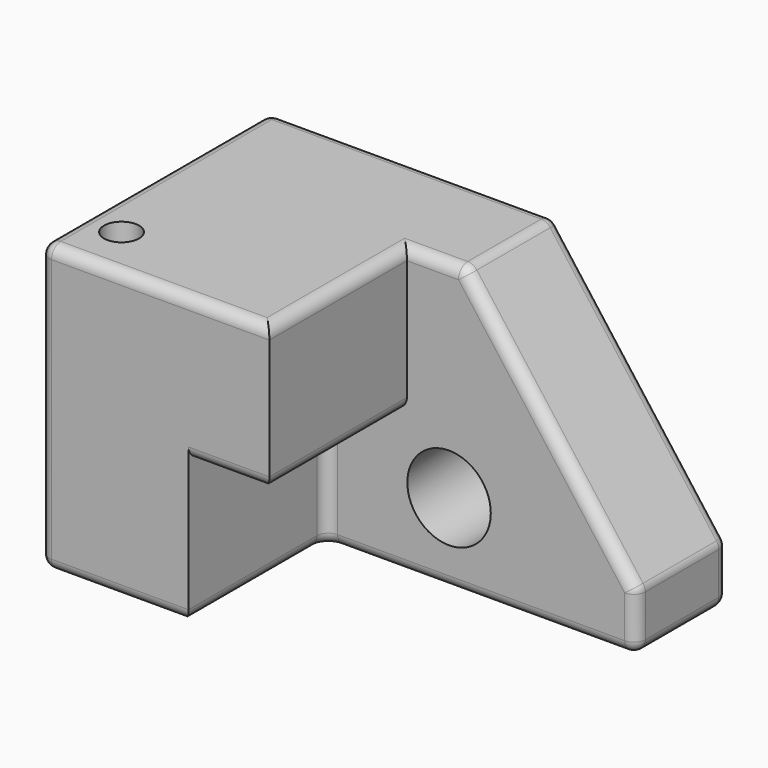
from build123d import *

# Parameters (mm, degrees)
F0_W         = 203.2
F0_H         = 127
F1_DEPTH     = 127
F3_DEPTH     = 76.2
F4_SIZE2     = 101.6
F4_SIZE      = 76.2
F5_R         = 5.08
F6_T1_DEPTH  = 116.84
F6_T3_DEPTH  = 116.84
F6_T5_DEPTH  = 193.04
F6_S9_W      = 5.08
F6_S9_H      = 5.08
F6_T10_DEPTH = 5.08
F6_S15_W     = 5.08
F6_S15_H     = 5.08
F6_T16_DEPTH = 5.08
F6_S21_W     = 5.08
F6_S21_H     = 5.08
F6_T22_DEPTH = 5.08
F6_S27_W     = 5.08
F6_S27_H     = 5.08
F6_T28_DEPTH = 5.08
F7_R         = 18.4939106261
F8_DEPTH     = 50.8
F9_R         = 7.7650869993
F10_DEPTH    = 127


# Not quite as in the source:
# - a fillet or chamfer that OpenCascade refuses, or shapes differently, is made with other operations: its cross-section is extruded or revolved along the edge and cut away or added


with BuildPart() as f1:
    # F0 (on Front) → F1 (new body)
    with BuildSketch(Plane.XZ):
        Rectangle(F0_W, F0_H)
    extrude(amount=F1_DEPTH)

    # F2 (on face) → F3 (cut)
    with BuildSketch(Plane.XZ.offset(127)):
        Polygon((101.6, 63.5), (0, 63.5), (0, 0), (-35.8415916562, 0), (-35.8415916562, -63.5), (101.6, -63.5), align=None)
    extrude(amount=-F3_DEPTH, mode=Mode.SUBTRACT)

    # F4
    f4_edges = [f1.edges().sort_by_distance(p)[0] for p in [
        (101.6, -25.4, 63.5),
    ]]
    f4_side = f1.faces().sort_by_distance((-21.771429, -52.614286, 63.5))[0]
    chamfer(f4_edges, length=F4_SIZE, length2=F4_SIZE2, reference=f4_side)

    # F5
    f5_edges = [f1.edges().sort_by_distance(p)[0] for p in [
        (-101.6, -63.5, 63.5),
        (-50.8, -127, 63.5),
        (0, -88.9, 63.5),
        (12.7, -50.8, 63.5),
        (25.4, -25.4, 63.5),
        (-38.1, 0, 63.5),
        (-17.920796, -127, 0),
        (0, -88.9, 0),
        (-101.6, -127, 0),
        (-68.720796, -127, -63.5),
        (-35.841592, -88.9, -63.5),
        (-35.841592, -50.8, -31.75),
        (32.879204, -50.8, -63.5),
        (101.6, -50.8, -50.8),
        (101.6, -25.4, -63.5),
        (101.6, 0, -50.8),
        (101.6, -25.4, -38.1),
        (63.5, -50.8, 12.7),
        (63.5, 0, 12.7),
    ]]
    fillet(f5_edges, radius=F5_R)

    # F6: fillet of radius 5.08 on 3 edges, made by hand

    # F6_s2 → F6_t1 (cut)
    with BuildSketch(Plane.XZ.offset(5.08)):
        with BuildLine():
            ThreePointArc((-96.52, -63.5), (-100.1121024484, -62.0121024484), (-101.6, -58.42))
            Line((-101.6, -58.42), (-101.6, -63.5))
            Line((-101.6, -63.5), (-96.52, -63.5))
        make_face()
    extrude(amount=F6_T1_DEPTH, mode=Mode.SUBTRACT)

    # F6_s4 → F6_t3 (cut)
    with BuildSketch(Plane.XY.offset(-58.42)):
        with BuildLine():
            ThreePointArc((-96.52, 0), (-100.1121024484, -1.4878975516), (-101.6, -5.08))
            Line((-101.6, -5.08), (-101.6, 0))
            Line((-101.6, 0), (-96.52, 0))
        make_face()
    extrude(amount=F6_T3_DEPTH, mode=Mode.SUBTRACT)

    # F6_s6 → F6_t5 (cut)
    with BuildSketch(Plane.YZ.offset(-96.52)):
        with BuildLine():
            ThreePointArc((0, -58.42), (-1.4878975516, -62.0121024484), (-5.08, -63.5))
            Line((-5.08, -63.5), (0, -63.5))
            Line((0, -63.5), (0, -58.42))
        make_face()
    extrude(amount=F6_T5_DEPTH, mode=Mode.SUBTRACT)


with BuildPart() as f6_tool8:
    # F6_s9 → F6_t10 (new body)
    with BuildSketch(Plane.XZ.offset(5.08)):
        with Locations((99.06, -60.96)):
            Rectangle(F6_S9_W, F6_S9_H)
    extrude(amount=-F6_T10_DEPTH)

    # F6_s11 → F6_t12 (revolve, cut)
    with BuildSketch(Plane(origin=(96.52, -5.08, -58.42), x_dir=(-0.7071067812, 0, 0.7071067812), z_dir=(-0.7071067812, 0, -0.7071067812))):
        with BuildLine():
            ThreePointArc((0, -5.08), (5.08, 0), (0, 5.08))
            Line((0, 5.08), (0, -5.08))
        make_face()
    revolve(axis=Axis((96.52, -5.08, -58.42), (0, 1, 0)), mode=Mode.SUBTRACT)


with BuildPart() as f1_1:
    add(f1.part)

    # F6_t7: cut F6_tool8
    add(f6_tool8.part, mode=Mode.SUBTRACT)


with BuildPart() as f6_tool14:
    # F6_s15 → F6_t16 (new body)
    with BuildSketch(Plane.XZ.offset(5.08)):
        with Locations((-99.06, 60.96)):
            Rectangle(F6_S15_W, F6_S15_H)
    extrude(amount=-F6_T16_DEPTH)

    # F6_s17 → F6_t18 (revolve, cut)
    with BuildSketch(Plane(origin=(-96.52, -5.08, 58.42), x_dir=(0.7071067812, 0, -0.7071067812), z_dir=(0.7071067812, 0, 0.7071067812))):
        with BuildLine():
            ThreePointArc((0, -5.08), (5.08, 0), (0, 5.08))
            Line((0, 5.08), (0, -5.08))
        make_face()
    revolve(axis=Axis((-96.52, -5.08, 58.42), (0, 1, 0)), mode=Mode.SUBTRACT)


with BuildPart() as f1_2:
    add(f1_1.part)

    # F6_t13: cut F6_tool14
    add(f6_tool14.part, mode=Mode.SUBTRACT)


with BuildPart() as f6_tool20:
    # F6_s21 → F6_t22 (new body)
    with BuildSketch(Plane.XY.offset(-58.42)):
        with Locations((-99.06, -124.46)):
            Rectangle(F6_S21_W, F6_S21_H)
    extrude(amount=-F6_T22_DEPTH)

    # F6_s23 → F6_t24 (revolve, cut)
    with BuildSketch(Plane(origin=(-96.52, -121.92, -58.42), x_dir=(0.7071067812, 0.7071067812, 0), z_dir=(-0.7071067812, 0.7071067812, 0))):
        with BuildLine():
            ThreePointArc((0, -5.08), (5.08, 0), (0, 5.08))
            Line((0, 5.08), (0, -5.08))
        make_face()
    revolve(axis=Axis((-96.52, -121.92, -58.42), (0, 0, -1)), mode=Mode.SUBTRACT)


with BuildPart() as f1_3:
    add(f1_2.part)

    # F6_t19: cut F6_tool20
    add(f6_tool20.part, mode=Mode.SUBTRACT)


with BuildPart() as f6_tool26:
    # F6_s27 → F6_t28 (new body)
    with BuildSketch(Plane.XZ.offset(5.08)):
        with Locations((-99.06, -60.96)):
            Rectangle(F6_S27_W, F6_S27_H)
    extrude(amount=-F6_T28_DEPTH)

    # F6_s29 → F6_t30 (revolve, cut)
    with BuildSketch(Plane(origin=(-96.52, -5.08, -58.42), x_dir=(0.7071067812, 0, 0.7071067812), z_dir=(-0.7071067812, 0, 0.7071067812))):
        with BuildLine():
            ThreePointArc((0, -5.08), (5.08, 0), (0, 5.08))
            Line((0, 5.08), (0, -5.08))
        make_face()
    revolve(axis=Axis((-96.52, -5.08, -58.42), (0, 1, 0)), mode=Mode.SUBTRACT)


with BuildPart() as f1_4:
    add(f1_3.part)

    # F6_t25: cut F6_tool26
    add(f6_tool26.part, mode=Mode.SUBTRACT)

    # F7 (on face) → F8 (cut, through all)
    with BuildSketch(Plane.XZ.offset(50.8)):
        with Locations((18.6727233231, -28.0290115625)):
            Circle(F7_R)
    extrude(amount=-F8_DEPTH, mode=Mode.SUBTRACT)

    # F9 (on face) → F10 (cut, through all)
    with BuildSketch(Plane.XY.offset(63.5)):
        with Locations((-84.4542831182, -103.3027470112)):
            Circle(F9_R)
    extrude(amount=-F10_DEPTH, mode=Mode.SUBTRACT)


solid = f1_4.part
